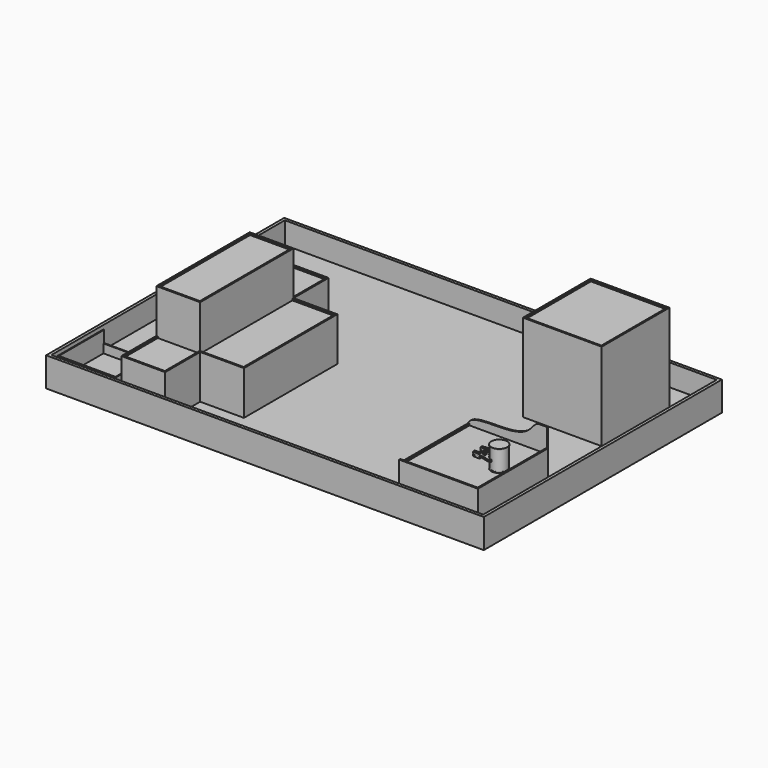
from build123d import *

# Parameters (mm, degrees)
F0_R      = 27.2
F1_DEPTH  = 2.83
F2_R      = 26.4
F3_DEPTH  = 67.36
F4_R      = 27.2
F5_DEPTH  = 2.83
F9_W      = 270
F9_H      = 300
F10_DEPTH = 72
F12_DEPTH = 15
F14_DEPTH = 5
F15_W     = 5
F15_H     = 290
F16_DEPTH = 5
F17_W     = 1500
F17_H     = 1020
F18_DEPTH = 25
F19_W     = 270
F19_H     = 290
F20_DEPTH = 300
F21_W     = 260
F21_H     = 280
F22_DEPTH = 5
F23_W     = 1500
F23_H     = 1020
F23_W_2   = 1480
F23_H_2   = 1000
F24_DEPTH = 75
F26_DEPTH = 150
F27_W     = 150
F27_H     = 400
F28_DEPTH = 150
F29_W     = 140
F29_H     = 390
F30_DEPTH = 5
F31_W     = 140
F31_H     = 145
F31_W_2   = 145
F31_H_2   = 390
F32_DEPTH = 5
F33_R     = 3
F34_DEPTH = 4
F35_R     = 3.99999
F35_2_R   = 3.99999
F36_R     = 3
F37_DEPTH = 8
F38_R     = 3
F39_DEPTH = 8
F40_R     = 3
F40_R_2   = 2.5
F41_DEPTH = 3
F42_R     = 3
F42_R_2   = 2.5
F43_DEPTH = 3
F45_DEPTH = 270.001
F46_W     = 200
F46_H     = 200
F46_W_2   = 194
F46_H_2   = 191
F47_DEPTH = 30
F49_DEPTH = 40
F50_R     = 2.5
F51_DEPTH = 5
F52_DEPTH = 6


# Not quite as in the source:
# - a fillet or chamfer is up to 0.001 mm smaller than in the source, because OpenCascade refuses the exact size
# - a feature names something its author has since deleted; it is built from what else it names


with BuildPart() as f1:
    # F0 (on Top) → F1 (new body)
    with BuildSketch(Plane.XY):
        Circle(F0_R)
    extrude(amount=F1_DEPTH)

    # F2 (on face) → F3 (join)
    with BuildSketch(Plane.XY.offset(2.83)):
        Circle(F2_R)
    extrude(amount=F3_DEPTH)

    # F4 (on face) → F5 (join)
    with BuildSketch(Plane.XY.offset(70.19)):
        Circle(F4_R)
    extrude(amount=F5_DEPTH)


with BuildPart() as f10:
    # F9 (on Top) → F10 (new body)
    with BuildSketch(Plane.XY):
        with Locations((-87.8, 0)):
            Rectangle(F9_W, F9_H)
    extrude(amount=-F10_DEPTH)

    # F11 (on face) → F12 (join)
    with BuildSketch(Plane.XY):
        Polygon((-222.8, -145), (-222.8, -150), (47.2, -150), (47.2, 150), (42.2, 150), (42.2, -145), align=None)
    extrude(amount=F12_DEPTH)

    # F13 (on face) → F14 (join)
    with BuildSketch(Plane(origin=(0, 150, 0), x_dir=(-1, 0, 0), z_dir=(0, 1, 0))):
        with BuildLine():
            Line((-21.3134280931, 81.3575685024), (-47.2, 81.3575685024))
            Line((-47.2, 81.3575685024), (-47.2, -72))
            Line((-47.2, -72), (222.8, -72))
            Line((222.8, -72), (222.8, 0))
            add(Edge.make_bspline(
                [(-21.3134280931, 81.3575685024), (-6.3059147253, 81.3822787863), (12.9585432644, 38.1268753575), (103.6097013063, 23.6068887567), (223.0224295336, 30.7718731823), (222.8, 0)],
                knots=[0, 0, 0, 0, 0.2487100673, 0.6151112321, 1, 1, 1, 1], degree=3))
        make_face()
    extrude(amount=-F14_DEPTH)

    # F15 (on face) → F16 (join)
    with BuildSketch(Plane.XY):
        with Locations((-220.3, 0)):
            Rectangle(F15_W, F15_H)
    extrude(amount=F16_DEPTH)

    # F17 (on face) → F18 (join)
    with BuildSketch(Plane(origin=(0, 0, -72), x_dir=(1, 0, 0), z_dir=(0, 0, -1))):
        with Locations((-602.8, -260)):
            Rectangle(F17_W, F17_H)
    extrude(amount=F18_DEPTH)

    # F19 (on face) → F20 (join)
    with BuildSketch(Plane.XY.offset(-72)):
        with Locations((-87.8, 525)):
            Rectangle(F19_W, F19_H)
    extrude(amount=F20_DEPTH)

    # F21 (on face) → F22 (cut)
    with BuildSketch(Plane.XY.offset(228)):
        with Locations((-87.8, 525)):
            Rectangle(F21_W, F21_H)
    extrude(amount=-F22_DEPTH, mode=Mode.SUBTRACT)

    # F23 (on face) → F24 (join)
    with BuildSketch(Plane.XY.offset(-72)):
        with Locations((-602.8, 260)):
            Rectangle(F23_W, F23_H)
        with Locations((-602.8, 260)):
            Rectangle(F23_W_2, F23_H_2, mode=Mode.SUBTRACT)
    extrude(amount=F24_DEPTH)

    # F25 (on face) → F26 (join)
    with BuildSketch(Plane.XY.offset(-72)):
        Polygon((-952.8, 460), (-1102.8, 460), (-1102.8, -240), (-952.8, -240), (-952.8, -90), (-802.8, -90), (-802.8, 310), (-952.8, 310), align=None)
    extrude(amount=F26_DEPTH)

    # F27 (on face) → F28 (join)
    with BuildSketch(Plane.XY.offset(78)):
        with Locations((-1027.8, 110)):
            Rectangle(F27_W, F27_H)
    extrude(amount=F28_DEPTH)

    # F29 (on face) → F30 (cut)
    with BuildSketch(Plane.XY.offset(228)):
        with Locations((-1027.8, 110)):
            Rectangle(F29_W, F29_H)
    extrude(amount=-F30_DEPTH, mode=Mode.SUBTRACT)

    # F31 (on face) → F32 (cut)
    with BuildSketch(Plane.XY.offset(78)):
        with Locations((-1027.8, 382.5)):
            Rectangle(F31_W, F31_H)
        with Locations((-880.3, 110)):
            Rectangle(F31_W_2, F31_H_2)
        with Locations((-1027.8, -162.5)):
            Rectangle(F31_W, F31_H)
    extrude(amount=-F32_DEPTH, mode=Mode.SUBTRACT)

    # F46 (on face) → F47 (join)
    with BuildSketch(Plane.XY.offset(-72)):
        with Locations((-1232.8, -130)):
            Rectangle(F46_W, F46_H)
        with Locations((-1232.8, -128.5)):
            Rectangle(F46_W_2, F46_H_2, mode=Mode.SUBTRACT)
    extrude(amount=F47_DEPTH)

    # F48 (on face) → F49 (join)
    with BuildSketch(Plane.XY.offset(-42)):
        Polygon((-1329.8, -30), (-1332.8, -30), (-1332.8, -230), (-1329.8, -230), (-1135.8, -230), (-1132.8, -230), (-1132.8, -30), (-1135.8, -30), (-1135.8, -224), (-1329.8, -224), align=None)
    extrude(amount=F49_DEPTH)


with BuildPart() as f34:
    # F33 (on offset) → F34 (new body, symmetric)
    with BuildSketch(Plane.XY.offset(25)):
        with BuildLine():
            Line((-55, -12), (-74.5, -12))
            Line((-74.5, -12), (-74.5, -13))
            Line((-74.5, -13), (-65.6457513111, -13))
            ThreePointArc((-65.6457513111, -13), (-67, -16), (-65.6457513111, -19))
            Line((-65.6457513111, -19), (-74.5, -19))
            Line((-74.5, -19), (-74.5, -20))
            Line((-74.5, -20), (-55, -20))
            ThreePointArc((-55, -20), (-51, -16), (-55, -12))
        make_face()
        with Locations((-63, -16)):
            Circle(F33_R, mode=Mode.SUBTRACT)
        with Locations((-55, -16)):
            Circle(F33_R, mode=Mode.SUBTRACT)
    extrude(amount=F34_DEPTH, both=True)

    # F35 (radius 4 in the source; OpenCascade refuses exactly that, so slightly less here)
    f35_edges = [f34.edges().sort_by_distance(p)[0] for p in [
        (-74.5, -19.5, 29),
        (-74.5, -12.5, 29),
        (-74.5, -19.5, 21),
        (-74.5, -12.5, 21),
    ]]
    fillet(f35_edges, radius=F35_R)

    # F36 (on face) → F37 (join, through all)
    with BuildSketch(Plane.XZ.offset(20)):
        with Locations((-70.5, 25)):
            Circle(F36_R)
    extrude(amount=-F37_DEPTH)

    # F42 (on offset) → F43 (join, symmetric)
    with BuildSketch(Plane.XY.offset(25)):
        with Locations((-63, -16)):
            Circle(F42_R)
        with Locations((-63, -16)):
            Circle(F42_R_2, mode=Mode.SUBTRACT)
        with Locations((-55, -16)):
            Circle(F42_R)
        with Locations((-55, -16)):
            Circle(F42_R_2, mode=Mode.SUBTRACT)
    extrude(amount=F43_DEPTH, both=True)


with BuildPart() as f34b:
    # F33 (on offset) → F34, piece 2 (new body, symmetric)
    with BuildSketch(Plane.XY.offset(25)):
        with BuildLine():
            Line((-74.5, 13), (-74.5, 12))
            Line((-74.5, 12), (-55, 12))
            ThreePointArc((-55, 12), (-51, 16), (-55, 20))
            Line((-55, 20), (-74.5, 20))
            Line((-74.5, 20), (-74.5, 19))
            Line((-74.5, 19), (-65.6457513111, 19))
            ThreePointArc((-65.6457513111, 19), (-67, 16), (-65.6457513111, 13))
            Line((-65.6457513111, 13), (-74.5, 13))
        make_face()
        with Locations((-63, 16)):
            Circle(F33_R, mode=Mode.SUBTRACT)
        with Locations((-55, 16)):
            Circle(F33_R, mode=Mode.SUBTRACT)
    extrude(amount=F34_DEPTH, both=True)

    # F35#2 (radius 4 in the source; OpenCascade refuses exactly that, so slightly less here)
    f35_2_edges = [f34b.edges().sort_by_distance(p)[0] for p in [
        (-74.5, 12.5, 29),
        (-74.5, 19.5, 29),
        (-74.5, 19.5, 21),
        (-74.5, 12.5, 21),
    ]]
    fillet(f35_2_edges, radius=F35_2_R)

    # F38 (on face) → F39 (join, through all)
    with BuildSketch(Plane(origin=(0, 20, 0), x_dir=(-1, 0, 0), z_dir=(0, 1, 0))):
        with Locations((70.5, 25)):
            Circle(F38_R)
    extrude(amount=-F39_DEPTH)

    # F40 (on offset) → F41 (join, symmetric)
    with BuildSketch(Plane.XY.offset(25)):
        with Locations((-55, 16)):
            Circle(F40_R)
        with Locations((-55, 16)):
            Circle(F40_R_2, mode=Mode.SUBTRACT)
        with Locations((-63, 16)):
            Circle(F40_R)
        with Locations((-63, 16)):
            Circle(F40_R_2, mode=Mode.SUBTRACT)
    extrude(amount=F41_DEPTH, both=True)


with BuildPart() as f45_tool:
    # F44 (on face) → F45 (new body, through all)
    with BuildSketch(Plane(origin=(0, 20, 0), x_dir=(-1, 0, 0), z_dir=(0, 1, 0))):
        with BuildLine():
            Line((71.5, 26), (71.5, 27.2912878475))
            ThreePointArc((71.5, 27.2912878475), (70.5, 27.5), (69.5, 27.2912878475))
            Line((69.5, 27.2912878475), (69.5, 26))
            Line((69.5, 26), (68.2087121525, 26))
            ThreePointArc((68.2087121525, 26), (68, 25), (68.2087121525, 24))
            Line((68.2087121525, 24), (69.5, 24))
            Line((69.5, 24), (69.5, 22.7087121525))
            ThreePointArc((69.5, 22.7087121525), (70.5, 22.5), (71.5, 22.7087121525))
            Line((71.5, 22.7087121525), (71.5, 24))
            Line((71.5, 24), (72.7912878475, 24))
            ThreePointArc((72.7912878475, 24), (73, 25), (72.7912878475, 26))
            Line((72.7912878475, 26), (71.5, 26))
        make_face()
    extrude(amount=-F45_DEPTH)


with BuildPart() as f34_1:
    add(f34.part)

    # F45: cut by f45_tool
    add(f45_tool.part, mode=Mode.SUBTRACT)


with BuildPart() as f34b_1:
    add(f34b.part)

    # F45: cut by f45_tool
    add(f45_tool.part, mode=Mode.SUBTRACT)


with BuildPart() as f51:
    # F50 (on face) → F51 (new body)
    with BuildSketch(Plane.XY.offset(29)):
        with BuildLine():
            add(Edge.make_bspline(
                [(-74.2329060821, 20), (-44.9317372951, 20.5015945062), (-20.0854547427, 31.9990841688), (-5.4796424043, 31.9990841688)],
                knots=[0, 0, 0, 0, 69.7924729985, 69.7924729985, 69.7924729985, 69.7924729985], degree=3))
            Line((-74.2329060821, 20), (-74.1977286978, 12))
            Line((-74.1977286978, 12), (-54.3867349625, 12))
            Line((-54.3867349625, 12), (-54.3867349625, 0))
            Line((-54.3867349625, 0), (-54.3867349625, -12))
            Line((-54.3867349625, -12), (-74.1977286978, -12))
            Line((-74.1977286978, -12), (-74.2329060821, -20))
            add(Edge.make_bspline(
                [(-74.2329060821, -20), (-44.9317372951, -20.5015945062), (-20.0854547427, -31.9990841688), (-5.4796424043, -31.9990841688)],
                knots=[0, 0, 0, 0, 69.7924729985, 69.7924729985, 69.7924729985, 69.7924729985], degree=3))
            Line((-5.4796424043, -31.9990841688), (-5.4561090459, -26.6471550842))
            ThreePointArc((-5.4561090459, -26.6471550842), (-19.2174555051, -19.2491403421), (-26.638130565, -5.5))
            Line((-26.638130565, -5.5), (-31.6020000234, -6.1))
            Line((-31.6020000234, -6.1), (-31.6020000234, 0))
            Line((-31.6020000234, 0), (-31.6020000234, 6.1))
            Line((-31.6020000234, 6.1), (-26.638130565, 5.5))
            ThreePointArc((-26.638130565, 5.5), (-19.2174555051, 19.2491403421), (-5.4561090459, 26.6471550842))
            Line((-5.4561090459, 26.6471550842), (-5.4796424043, 31.9990841688))
        make_face()
        with Locations((-63, -16)):
            Circle(F50_R, mode=Mode.SUBTRACT)
        with Locations((-55, -16)):
            Circle(F50_R, mode=Mode.SUBTRACT)
        with BuildLine():
            add(Edge.make_bspline(
                [(-49.2716804147, 0), (-50.4164208351, -3.5035182948), (-52.9410664802, -11.2302850339), (-29.0629828433, -22.6522577332), (-37.0350109676, -7.7636960082), (-41.1920547485, 0)],
                knots=[0, 0, 0, 0, 0.28417626, 0.6267310425, 1, 1, 1, 1], degree=3))
            add(Edge.make_bspline(
                [(-49.2716804147, 0), (-50.4164208351, 3.5035182948), (-52.9410664802, 11.2302850339), (-29.0629828433, 22.6522577332), (-37.0350109676, 7.7636960082), (-41.1920547485, 0)],
                knots=[0, 0, 0, 0, 0.28417626, 0.6267310425, 1, 1, 1, 1], degree=3))
        make_face(mode=Mode.SUBTRACT)
        with Locations((-63, 16)):
            Circle(F50_R, mode=Mode.SUBTRACT)
        with Locations((-55, 16)):
            Circle(F50_R, mode=Mode.SUBTRACT)
    extrude(amount=F51_DEPTH)

    # F50 (on face) → F52 (join)
    with BuildSketch(Plane.XY.offset(29)):
        with BuildLine():
            add(Edge.make_bspline(
                [(-74.2329060821, 20), (-44.9317372951, 20.5015945062), (-20.0854547427, 31.9990841688), (-5.4796424043, 31.9990841688)],
                knots=[0, 0, 0, 0, 69.7924729985, 69.7924729985, 69.7924729985, 69.7924729985], degree=3))
            Line((-74.2329060821, 20), (-74.1977286978, 12))
            Line((-74.1977286978, 12), (-54.3867349625, 12))
            Line((-54.3867349625, 12), (-54.3867349625, 0))
            Line((-54.3867349625, 0), (-54.3867349625, -12))
            Line((-54.3867349625, -12), (-74.1977286978, -12))
            Line((-74.1977286978, -12), (-74.2329060821, -20))
            add(Edge.make_bspline(
                [(-74.2329060821, -20), (-44.9317372951, -20.5015945062), (-20.0854547427, -31.9990841688), (-5.4796424043, -31.9990841688)],
                knots=[0, 0, 0, 0, 69.7924729985, 69.7924729985, 69.7924729985, 69.7924729985], degree=3))
            Line((-5.4796424043, -31.9990841688), (-5.4561090459, -26.6471550842))
            ThreePointArc((-5.4561090459, -26.6471550842), (-19.2174555051, -19.2491403421), (-26.638130565, -5.5))
            Line((-26.638130565, -5.5), (-31.6020000234, -6.1))
            Line((-31.6020000234, -6.1), (-31.6020000234, 0))
            Line((-31.6020000234, 0), (-31.6020000234, 6.1))
            Line((-31.6020000234, 6.1), (-26.638130565, 5.5))
            ThreePointArc((-26.638130565, 5.5), (-19.2174555051, 19.2491403421), (-5.4561090459, 26.6471550842))
            Line((-5.4561090459, 26.6471550842), (-5.4796424043, 31.9990841688))
        make_face()
        with Locations((-63, -16)):
            Circle(F50_R, mode=Mode.SUBTRACT)
        with Locations((-55, -16)):
            Circle(F50_R, mode=Mode.SUBTRACT)
        with BuildLine():
            add(Edge.make_bspline(
                [(-49.2716804147, 0), (-50.4164208351, -3.5035182948), (-52.9410664802, -11.2302850339), (-29.0629828433, -22.6522577332), (-37.0350109676, -7.7636960082), (-41.1920547485, 0)],
                knots=[0, 0, 0, 0, 0.28417626, 0.6267310425, 1, 1, 1, 1], degree=3))
            add(Edge.make_bspline(
                [(-49.2716804147, 0), (-50.4164208351, 3.5035182948), (-52.9410664802, 11.2302850339), (-29.0629828433, 22.6522577332), (-37.0350109676, 7.7636960082), (-41.1920547485, 0)],
                knots=[0, 0, 0, 0, 0.28417626, 0.6267310425, 1, 1, 1, 1], degree=3))
        make_face(mode=Mode.SUBTRACT)
        with Locations((-63, 16)):
            Circle(F50_R, mode=Mode.SUBTRACT)
        with Locations((-55, 16)):
            Circle(F50_R, mode=Mode.SUBTRACT)
    extrude(amount=F52_DEPTH)


solid = Compound([f1.part, f10.part, f34_1.part, f34b_1.part, f51.part])
